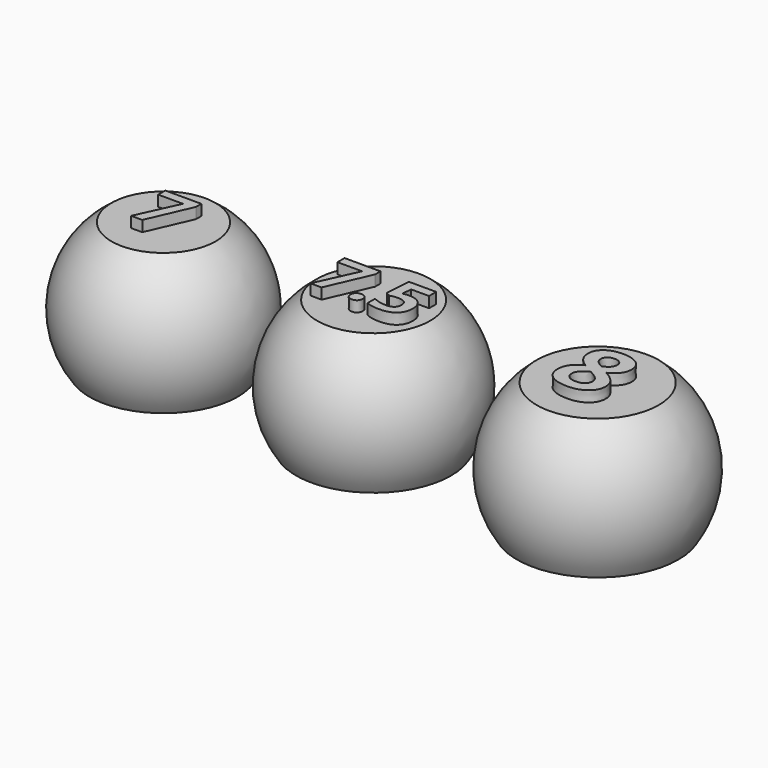
from build123d import *

# Parameters (mm, degrees)
F4_TEXT_SIZE = 6.5106313236
F5_DEPTH     = 1
F6_TEXT_SIZE = 6.4955234442
F7_DEPTH     = 1
F8_TEXT_SIZE = 8.8485591631
F9_DEPTH     = 1


# Not quite as in the source:
# - Text() gives the source's letters only with a copy of the font that has no kerning and outlines rounded to 1/6400 em; it was checked with that copy


with BuildPart() as f1:
    # F0 (on Front) → F1 (revolve)
    with BuildSketch(Plane.XZ):
        with BuildLine():
            Line((-40.2126908302, 0), (-33.3388272878, 0))
            ThreePointArc((-33.3388272878, 0), (-31.8344958877, 6.4338233872), (-35.3926927056, 12.0012583211))
            Line((-35.3926927056, 12.0012583211), (-40.2126908302, 12.0012583211))
            Line((-40.2126908302, 12.0012583211), (-40.2126908302, 0))
        make_face()
    revolve(axis=Axis((-40.2126908302, 0, 6.0006291606), (0, 0, -1)))

    # F4 (on face) → F5 (join)
    with BuildSketch(Plane.XY.offset(12.0012583211)):
        with Locations((-42.1813838184, -2.1871948848)):
            Text('7', F4_TEXT_SIZE, font='Open Sans', font_style=FontStyle.BOLD, text_align=(TextAlign.LEFT, TextAlign.BOTTOM))
    extrude(amount=F5_DEPTH)


with BuildPart() as f2:
    # F0 (on Front) → F2 (revolve)
    with BuildSketch(Plane.XZ):
        with BuildLine():
            Line((-15.5028005658, 12.0012583211), (-20.7511223853, 12.0012583211))
            Line((-20.7511223853, 12.0012583211), (-20.7511223853, 0))
            Line((-20.7511223853, 0), (-13.5704190771, 0))
            ThreePointArc((-13.5704190771, 0), (-12.1123888711, 6.3909648706), (-15.5028005658, 12.0012583211))
        make_face()
    revolve(axis=Axis((-20.7511223853, 0, 6.0006291606), (0, 0, 1)))

    # F6 (on face) → F7 (join)
    with BuildSketch(Plane.XY.offset(12.0012583211)):
        with Locations((-25.4499791263, -2.3389087808)):
            Text('7.5', F6_TEXT_SIZE, font='Open Sans', font_style=FontStyle.BOLD, text_align=(TextAlign.LEFT, TextAlign.BOTTOM))
    extrude(amount=F7_DEPTH)


with BuildPart() as f3:
    # F0 (on Front) → F3 (revolve)
    with BuildSketch(Plane.XZ):
        with BuildLine():
            Line((5.6552968022, 12.0012583211), (0, 12.0012583211))
            Line((0, 12.0012583211), (0, 0))
            Line((0, 0), (7.4833147735, 0))
            ThreePointArc((7.4833147735, 0), (8.8973776393, 6.3552384081), (5.6552968022, 12.0012583211))
        make_face()
    revolve(axis=Axis((0, 0, 6.0006291606), (0, 0, 1)))

    # F8 (on face) → F9 (join)
    with BuildSketch(Plane.XY.offset(12.0012583211)):
        with Locations((-2.6993260253, -3.2413133886)):
            Text('8', F8_TEXT_SIZE, font='Open Sans', font_style=FontStyle.BOLD, text_align=(TextAlign.LEFT, TextAlign.BOTTOM))
    extrude(amount=F9_DEPTH)


solid = Compound([f1.part, f2.part, f3.part])
